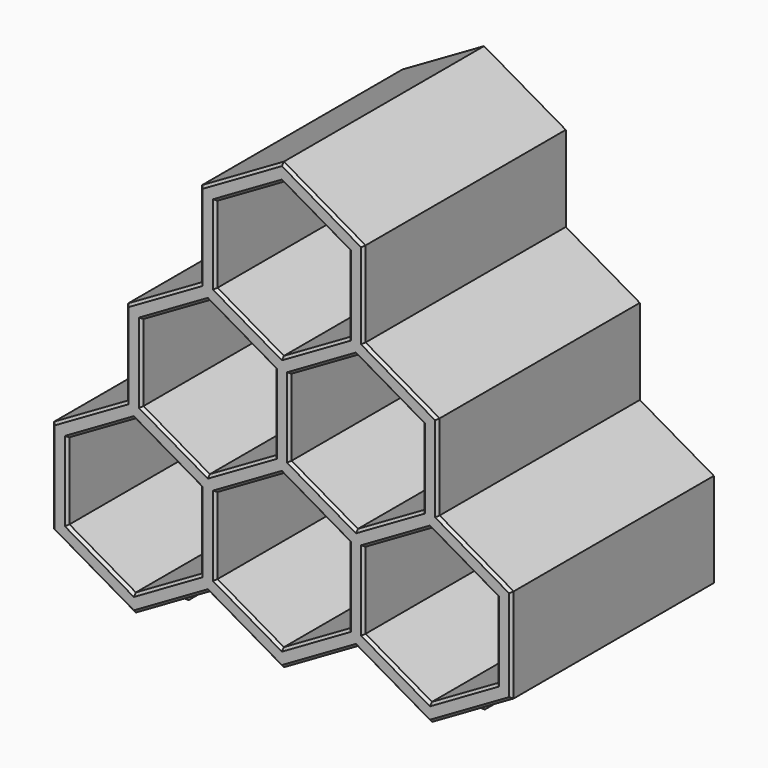
from build123d import *

# Parameters (mm, degrees)
F1_DEPTH      = 100
F22_W         = 15
F22_H         = 25
F23_DEPTH     = 5
F24_T4_DEPTH  = 20.3584149398
F24_T9_DEPTH  = 20.3584149398
F24_T14_DEPTH = 20.3584149398
F24_T19_DEPTH = 20.3584149398
F24_T24_DEPTH = 20.3584149398
F24_T29_DEPTH = 20.3584149398
F24_T34_DEPTH = 20.3584149398
F24_T39_DEPTH = 20.3584149398
F24_T44_DEPTH = 20.3584149398
F24_T49_DEPTH = 20.3584149398
F24_T54_DEPTH = 20.3584149398
F24_T59_DEPTH = 20.3584149398
F24_T64_DEPTH = 20.3584149398
F24_T69_DEPTH = 20.3584149398
F24_T74_DEPTH = 20.3584149398
F24_T79_DEPTH = 20.3584149398
F25_SIZE      = 1


# Not quite as in the source:
# - a fillet or chamfer that OpenCascade refuses, or shapes differently, is made with other operations: its cross-section is extruded or revolved along the edge and cut away or added


with BuildPart() as f1:
    # F0 (on Front) → F1 (new body)
    with BuildSketch(Plane.XZ):
        Polygon((32, -18.4752086141), (32, 18.4752086141), (0, 36.9504172281), (-32, 18.4752086141), (-32, -18.4752086141), (0, -36.9504172281), align=None)
        Polygon((0, 30.0222139979), (26, 15.0111069989), (26, -15.0111069989), (0, -30.0222139979), (-26, -15.0111069989), (-26, 15.0111069989), align=None, mode=Mode.SUBTRACT)
    extrude(amount=F1_DEPTH)


with BuildPart() as f4_1:
    # F4: copy of F1
    add(f1.part.moved(Location((58, 0, 0))))


with BuildPart() as f7_1:
    # F7: copy of F1
    add(f1.part.moved(Location((116, 0, 0))))


with BuildPart() as f10_1:
    # F10: copy of F1
    add(f1.part.moved(Location((29, 0, 50.2294734195))))


with BuildPart() as f13_1:
    # F13: copy of F1
    add(f1.part.moved(Location((87, 0, 50.2294734195))))


with BuildPart() as f16_1:
    # F16: copy of F1
    add(f1.part.moved(Location((58, 0, 100.458946839))))


with BuildPart() as f1_1:
    add(f1.part)

    # F17: union F10_1, F16_1, F4_1, F13_1, F7_1
    add(f10_1.part)
    add(f16_1.part)
    add(f4_1.part)
    add(f13_1.part)
    add(f7_1.part)


with BuildPart() as f1_2:
    # F20: moved
    add(f1_1.part.moved(Location((-58, 0, 0))))


with BuildPart() as f1_3:
    # F21: moved
    add(f1_2.part.moved(Location((0, 0, 36.9504172281))))

    # F22 (on Top) → F23 (join)
    with BuildSketch(Plane.XY):
        with Locations((-58, -75)):
            Rectangle(F22_W, F22_H)
        with Locations((58, -75)):
            Rectangle(F22_W, F22_H)
        with Locations((58, -25)):
            Rectangle(F22_W, F22_H)
        with Locations((-58, -25)):
            Rectangle(F22_W, F22_H)
    extrude(amount=F23_DEPTH)

    # F24: chamfer of 5 on 16 edges, made by hand


with BuildPart() as f24_tool2:
    # F24_s3 → F24_t4 (new body)
    with BuildSketch(Plane.YZ.offset(-78.3584149398)):
        Polygon((-37.5, 5), (-32.5, 0), (-37.5, 0), align=None)
    extrude(amount=F24_T4_DEPTH)

    split(bisect_by=Plane(origin=(-14.5, 0, -25.1147367097), x_dir=(0, 1, 0), z_dir=(-0.5, 0, -0.8660254038)), keep=Keep.TOP)


with BuildPart() as f1_4:
    add(f1_3.part)

    # F24_t1: cut F24_tool2
    add(f24_tool2.part, mode=Mode.SUBTRACT)


with BuildPart() as f24_tool7:
    # F24_s8 → F24_t9 (new body)
    with BuildSketch(Plane.YZ.offset(-58)):
        Polygon((-37.5, 5), (-32.5, 0), (-37.5, 0), align=None)
    extrude(amount=F24_T9_DEPTH)

    split(bisect_by=Plane(origin=(-14.5, 0, 25.1147367097), x_dir=(0, 1, 0), z_dir=(0.5, 0, -0.8660254038)), keep=Keep.TOP)


with BuildPart() as f1_5:
    add(f1_4.part)

    # F24_t6: cut F24_tool7
    add(f24_tool7.part, mode=Mode.SUBTRACT)


with BuildPart() as f24_tool12:
    # F24_s13 → F24_t14 (new body)
    with BuildSketch(Plane.YZ.offset(-58)):
        Polygon((-12.5, 5), (-17.5, 0), (-12.5, 0), align=None)
    extrude(amount=-F24_T14_DEPTH)

    split(bisect_by=Plane(origin=(-14.5, 0, -25.1147367097), x_dir=(0, 1, 0), z_dir=(-0.5, 0, -0.8660254038)), keep=Keep.TOP)


with BuildPart() as f1_6:
    add(f1_5.part)

    # F24_t11: cut F24_tool12
    add(f24_tool12.part, mode=Mode.SUBTRACT)


with BuildPart() as f24_tool17:
    # F24_s18 → F24_t19 (new body)
    with BuildSketch(Plane.YZ.offset(-37.6415850602)):
        Polygon((-12.5, 5), (-17.5, 0), (-12.5, 0), align=None)
    extrude(amount=-F24_T19_DEPTH)

    split(bisect_by=Plane(origin=(-14.5, 0, 25.1147367097), x_dir=(0, 1, 0), z_dir=(0.5, 0, -0.8660254038)), keep=Keep.TOP)


with BuildPart() as f1_7:
    add(f1_6.part)

    # F24_t16: cut F24_tool17
    add(f24_tool17.part, mode=Mode.SUBTRACT)


with BuildPart() as f24_tool22:
    # F24_s23 → F24_t24 (new body)
    with BuildSketch(Plane.YZ.offset(-58)):
        Polygon((-62.5, 5), (-67.5, 0), (-62.5, 0), align=None)
    extrude(amount=-F24_T24_DEPTH)

    split(bisect_by=Plane(origin=(-14.5, 0, -25.1147367097), x_dir=(0, 1, 0), z_dir=(-0.5, 0, -0.8660254038)), keep=Keep.TOP)


with BuildPart() as f1_8:
    add(f1_7.part)

    # F24_t21: cut F24_tool22
    add(f24_tool22.part, mode=Mode.SUBTRACT)


with BuildPart() as f24_tool27:
    # F24_s28 → F24_t29 (new body)
    with BuildSketch(Plane.YZ.offset(-37.6415850602)):
        Polygon((-62.5, 5), (-67.5, 0), (-62.5, 0), align=None)
    extrude(amount=-F24_T29_DEPTH)

    split(bisect_by=Plane(origin=(-14.5, 0, 25.1147367097), x_dir=(0, 1, 0), z_dir=(0.5, 0, -0.8660254038)), keep=Keep.TOP)


with BuildPart() as f1_9:
    add(f1_8.part)

    # F24_t26: cut F24_tool27
    add(f24_tool27.part, mode=Mode.SUBTRACT)


with BuildPart() as f24_tool32:
    # F24_s33 → F24_t34 (new body)
    with BuildSketch(Plane.YZ.offset(-78.3584149398)):
        Polygon((-87.5, 5), (-82.5, 0), (-87.5, 0), align=None)
    extrude(amount=F24_T34_DEPTH)

    split(bisect_by=Plane(origin=(-14.5, 0, -25.1147367097), x_dir=(0, 1, 0), z_dir=(-0.5, 0, -0.8660254038)), keep=Keep.TOP)


with BuildPart() as f1_10:
    add(f1_9.part)

    # F24_t31: cut F24_tool32
    add(f24_tool32.part, mode=Mode.SUBTRACT)


with BuildPart() as f24_tool37:
    # F24_s38 → F24_t39 (new body)
    with BuildSketch(Plane.YZ.offset(-58)):
        Polygon((-87.5, 5), (-82.5, 0), (-87.5, 0), align=None)
    extrude(amount=F24_T39_DEPTH)

    split(bisect_by=Plane(origin=(-14.5, 0, 25.1147367097), x_dir=(0, 1, 0), z_dir=(0.5, 0, -0.8660254038)), keep=Keep.TOP)


with BuildPart() as f1_11:
    add(f1_10.part)

    # F24_t36: cut F24_tool37
    add(f24_tool37.part, mode=Mode.SUBTRACT)


with BuildPart() as f24_tool42:
    # F24_s43 → F24_t44 (new body)
    with BuildSketch(Plane.YZ.offset(37.6415850602)):
        Polygon((-87.5, 5), (-82.5, 0), (-87.5, 0), align=None)
    extrude(amount=F24_T44_DEPTH)

    split(bisect_by=Plane(origin=(14.5, 0, 25.1147367097), x_dir=(0, 1, 0), z_dir=(-0.5, 0, -0.8660254038)), keep=Keep.TOP)


with BuildPart() as f1_12:
    add(f1_11.part)

    # F24_t41: cut F24_tool42
    add(f24_tool42.part, mode=Mode.SUBTRACT)


with BuildPart() as f24_tool47:
    # F24_s48 → F24_t49 (new body)
    with BuildSketch(Plane.YZ.offset(58)):
        Polygon((-87.5, 5), (-82.5, 0), (-87.5, 0), align=None)
    extrude(amount=F24_T49_DEPTH)

    split(bisect_by=Plane(origin=(14.5, 0, -25.1147367097), x_dir=(0, 1, 0), z_dir=(0.5, 0, -0.8660254038)), keep=Keep.TOP)


with BuildPart() as f1_13:
    add(f1_12.part)

    # F24_t46: cut F24_tool47
    add(f24_tool47.part, mode=Mode.SUBTRACT)


with BuildPart() as f24_tool52:
    # F24_s53 → F24_t54 (new body)
    with BuildSketch(Plane.YZ.offset(58)):
        Polygon((-62.5, 5), (-67.5, 0), (-62.5, 0), align=None)
    extrude(amount=-F24_T54_DEPTH)

    split(bisect_by=Plane(origin=(14.5, 0, 25.1147367097), x_dir=(0, 1, 0), z_dir=(-0.5, 0, -0.8660254038)), keep=Keep.TOP)


with BuildPart() as f1_14:
    add(f1_13.part)

    # F24_t51: cut F24_tool52
    add(f24_tool52.part, mode=Mode.SUBTRACT)


with BuildPart() as f24_tool57:
    # F24_s58 → F24_t59 (new body)
    with BuildSketch(Plane.YZ.offset(78.3584149398)):
        Polygon((-62.5, 5), (-67.5, 0), (-62.5, 0), align=None)
    extrude(amount=-F24_T59_DEPTH)

    split(bisect_by=Plane(origin=(14.5, 0, -25.1147367097), x_dir=(0, 1, 0), z_dir=(0.5, 0, -0.8660254038)), keep=Keep.TOP)


with BuildPart() as f1_15:
    add(f1_14.part)

    # F24_t56: cut F24_tool57
    add(f24_tool57.part, mode=Mode.SUBTRACT)


with BuildPart() as f24_tool62:
    # F24_s63 → F24_t64 (new body)
    with BuildSketch(Plane.YZ.offset(37.6415850602)):
        Polygon((-37.5, 5), (-32.5, 0), (-37.5, 0), align=None)
    extrude(amount=F24_T64_DEPTH)

    split(bisect_by=Plane(origin=(14.5, 0, 25.1147367097), x_dir=(0, 1, 0), z_dir=(-0.5, 0, -0.8660254038)), keep=Keep.TOP)


with BuildPart() as f1_16:
    add(f1_15.part)

    # F24_t61: cut F24_tool62
    add(f24_tool62.part, mode=Mode.SUBTRACT)


with BuildPart() as f24_tool67:
    # F24_s68 → F24_t69 (new body)
    with BuildSketch(Plane.YZ.offset(58)):
        Polygon((-37.5, 5), (-32.5, 0), (-37.5, 0), align=None)
    extrude(amount=F24_T69_DEPTH)

    split(bisect_by=Plane(origin=(14.5, 0, -25.1147367097), x_dir=(0, 1, 0), z_dir=(0.5, 0, -0.8660254038)), keep=Keep.TOP)


with BuildPart() as f1_17:
    add(f1_16.part)

    # F24_t66: cut F24_tool67
    add(f24_tool67.part, mode=Mode.SUBTRACT)


with BuildPart() as f24_tool72:
    # F24_s73 → F24_t74 (new body)
    with BuildSketch(Plane.YZ.offset(58)):
        Polygon((-12.5, 5), (-17.5, 0), (-12.5, 0), align=None)
    extrude(amount=-F24_T74_DEPTH)

    split(bisect_by=Plane(origin=(14.5, 0, 25.1147367097), x_dir=(0, 1, 0), z_dir=(-0.5, 0, -0.8660254038)), keep=Keep.TOP)


with BuildPart() as f1_18:
    add(f1_17.part)

    # F24_t71: cut F24_tool72
    add(f24_tool72.part, mode=Mode.SUBTRACT)


with BuildPart() as f24_tool77:
    # F24_s78 → F24_t79 (new body)
    with BuildSketch(Plane.YZ.offset(78.3584149398)):
        Polygon((-12.5, 5), (-17.5, 0), (-12.5, 0), align=None)
    extrude(amount=-F24_T79_DEPTH)

    split(bisect_by=Plane(origin=(14.5, 0, -25.1147367097), x_dir=(0, 1, 0), z_dir=(0.5, 0, -0.8660254038)), keep=Keep.TOP)


with BuildPart() as f1_19:
    add(f1_18.part)

    # F24_t76: cut F24_tool77
    add(f24_tool77.part, mode=Mode.SUBTRACT)

    # F25
    f25_edges = [f1_19.edges().sort_by_distance(p)[0] for p in [
        (-32, 0, 36.950417),
        (-45, 0, 14.433757),
        (-71, 0, 14.433757),
        (-84, 0, 36.950417),
        (-71, 0, 59.467078),
        (-45, 0, 59.467078),
        (-42, 0, 64.66323),
        (-55, 0, 87.179891),
        (-42, 0, 109.696551),
        (-16, 0, 109.696551),
        (-3, 0, 87.179891),
        (-16, 0, 64.66323),
        (-26, 0, 36.950417),
        (-13, 0, 59.467078),
        (13, 0, 59.467078),
        (26, 0, 36.950417),
        (13, 0, 14.433757),
        (-13, 0, 14.433757),
        (42, 0, 109.696551),
        (55, 0, 87.179891),
        (42, 0, 64.66323),
        (16, 0, 64.66323),
        (3, 0, 87.179891),
        (16, 0, 109.696551),
        (-61, 0, 88.911941),
        (-75.5, 0, 63.797205),
        (-90, 0, 36.950417),
        (-74, 0, 9.237604),
        (-43.5, 0, 8.371579),
        (-14.5, 0, 8.371579),
        (14.5, 0, 8.371579),
        (43.5, 0, 8.371579),
        (74, 0, 9.237604),
        (90, 0, 36.950417),
        (75.5, 0, 63.797205),
        (61, 0, 88.911941),
        (46.5, 0, 114.026678),
        (32, 0, 139.141415),
        (16, 0, 165.122177),
        (-16, 0, 165.122177),
        (-32, 0, 139.141415),
        (-46.5, 0, 114.026678),
        (32, 0, 36.950417),
        (45, 0, 59.467078),
        (71, 0, 59.467078),
        (84, 0, 36.950417),
        (71, 0, 14.433757),
        (45, 0, 14.433757),
        (26, 0, 137.409364),
        (13, 0, 114.892704),
        (-13, 0, 114.892704),
        (-26, 0, 137.409364),
        (-13, 0, 159.926025),
        (13, 0, 159.926025),
        (-32, -100, 36.950417),
        (-45, -100, 14.433757),
        (-71, -100, 14.433757),
        (-84, -100, 36.950417),
        (-71, -100, 59.467078),
        (-45, -100, 59.467078),
        (-42, -100, 64.66323),
        (-55, -100, 87.179891),
        (-42, -100, 109.696551),
        (-16, -100, 109.696551),
        (-3, -100, 87.179891),
        (-16, -100, 64.66323),
        (-26, -100, 36.950417),
        (-13, -100, 59.467078),
        (13, -100, 59.467078),
        (26, -100, 36.950417),
        (13, -100, 14.433757),
        (-13, -100, 14.433757),
        (42, -100, 109.696551),
        (55, -100, 87.179891),
        (42, -100, 64.66323),
        (16, -100, 64.66323),
        (3, -100, 87.179891),
        (16, -100, 109.696551),
        (-61, -100, 88.911941),
        (-75.5, -100, 63.797205),
        (-90, -100, 36.950417),
        (-74, -100, 9.237604),
        (-43.5, -100, 8.371579),
        (-14.5, -100, 8.371579),
        (14.5, -100, 8.371579),
        (43.5, -100, 8.371579),
        (74, -100, 9.237604),
        (90, -100, 36.950417),
        (75.5, -100, 63.797205),
        (61, -100, 88.911941),
        (46.5, -100, 114.026678),
        (32, -100, 139.141415),
        (16, -100, 165.122177),
        (-16, -100, 165.122177),
        (-32, -100, 139.141415),
        (-46.5, -100, 114.026678),
        (32, -100, 36.950417),
        (45, -100, 59.467078),
        (71, -100, 59.467078),
        (84, -100, 36.950417),
        (71, -100, 14.433757),
        (45, -100, 14.433757),
        (26, -100, 137.409364),
        (13, -100, 114.892704),
        (-13, -100, 114.892704),
        (-26, -100, 137.409364),
        (-13, -100, 159.926025),
        (13, -100, 159.926025),
    ]]
    chamfer(f25_edges, length=F25_SIZE)


solid = f1_19.part
